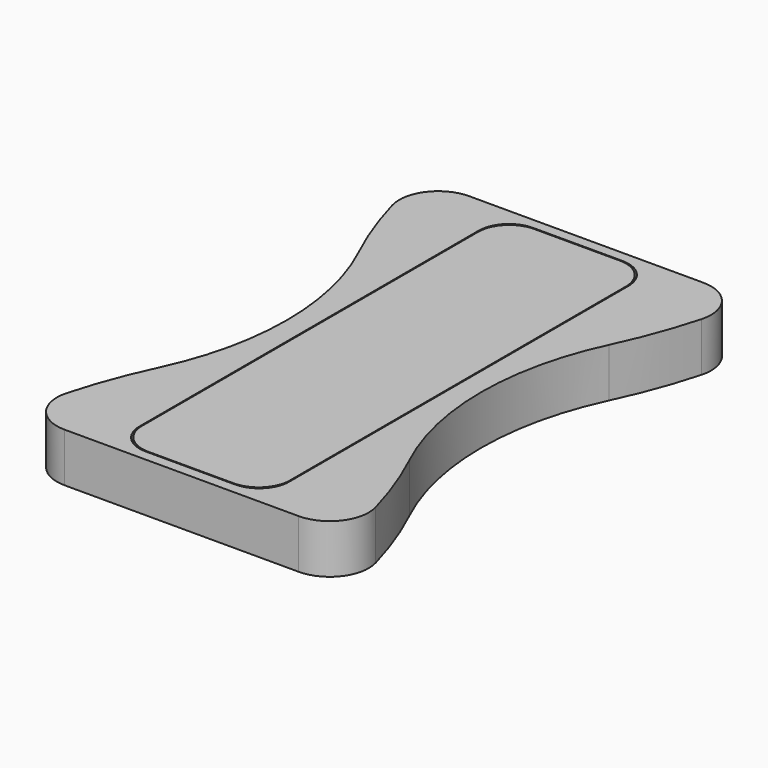
from build123d import *

# Parameters (mm, degrees)
F0_W         = 38
F0_H         = 124
F1_DEPTH     = 6.3
F2_R         = 8
F3_R         = 3
F5_DEPTH     = 6.3
F6_W         = 38.5
F6_H         = 124.5
F7_DEPTH     = 6.15
F8_R         = 7.75
F9_R         = 2.75
F11_DEPTH    = 12.601
F12_T1_DEPTH = 108.1589008266
F13_R        = 10


# Not quite as in the source:
# - a fillet or chamfer that OpenCascade refuses, or shapes differently, is made with other operations: its cross-section is extruded or revolved along the edge and cut away or added


with BuildPart() as f1:
    # F0 (on Top) → F1 (new body)
    with BuildSketch(Plane.XY):
        Rectangle(F0_W, F0_H)
    extrude(amount=F1_DEPTH)

    # F2
    f2_edges = [f1.edges().sort_by_distance(p)[0] for p in [
        (19, 62, 3.15),
        (-19, 62, 3.15),
        (19, -62, 3.15),
        (-19, -62, 3.15),
    ]]
    fillet(f2_edges, radius=F2_R)

    # F3
    f3_edges = [f1.edges().sort_by_distance(p)[0] for p in [
        (0, -62, 0),
        (-16.656854, -59.656854, 0),
        (16.656854, -59.656854, 0),
        (-19, 0, 0),
        (19, 0, 0),
        (-16.656854, 59.656854, 0),
        (16.656854, 59.656854, 0),
        (0, 62, 0),
    ]]
    fillet(f3_edges, radius=F3_R)


with BuildPart() as f5:
    # F4 (on Top) → F5 (new body, symmetric)
    with BuildSketch(Plane.XY):
        with BuildLine():
            Line((19.25, -27.1095328612), (19.25, -62.25))
            Line((19.25, -62.25), (-19.25, -62.25))
            Line((-19.25, -62.25), (-19.25, -27.1095328612))
            ThreePointArc((-19.25, -27.1095328612), (-36.224128699, -42.7724832696), (-42.5, -65))
            Line((-42.5, -65), (42.5, -65))
            ThreePointArc((42.5, -65), (36.224128699, -42.7724832696), (19.25, -27.1095328612))
        make_face()
        with BuildLine():
            ThreePointArc((-42.5, -65), (-36.224128699, -42.7724832696), (-19.25, -27.1095328612))
            Line((-19.25, -27.1095328612), (-19.25, 27.1095328612))
            ThreePointArc((-19.25, 27.1095328612), (-36.224128699, 42.7724832696), (-42.5, 65))
            Line((-42.5, 65), (-42.5, -65))
        make_face()
        with BuildLine():
            Line((19.25, 27.1095328612), (19.25, -27.1095328612))
            ThreePointArc((19.25, -27.1095328612), (36.224128699, -42.7724832696), (42.5, -65))
            Line((42.5, -65), (42.5, 65))
            ThreePointArc((42.5, 65), (36.224128699, 42.7724832696), (19.25, 27.1095328612))
        make_face()
        with BuildLine():
            Line((19.25, 62.25), (19.25, 27.1095328612))
            ThreePointArc((19.25, 27.1095328612), (36.224128699, 42.7724832696), (42.5, 65))
            Line((42.5, 65), (-42.5, 65))
            ThreePointArc((-42.5, 65), (-36.224128699, 42.7724832696), (-19.25, 27.1095328612))
            Line((-19.25, 27.1095328612), (-19.25, 62.25))
            Line((-19.25, 62.25), (19.25, 62.25))
        make_face()
    extrude(amount=F5_DEPTH, both=True)

    # F6 (on face) → F7 (join)
    with BuildSketch(Plane(origin=(0, 0, -6.3), x_dir=(1, 0, 0), z_dir=(0, 0, -1))):
        Rectangle(F6_W, F6_H)
    extrude(amount=-F7_DEPTH)

    # F8
    f8_edges = [f5.edges().sort_by_distance(p)[0] for p in [
        (19.25, -62.25, 3.075),
        (-19.25, -62.25, 3.075),
        (19.25, 62.25, 3.075),
        (-19.25, 62.25, 3.075),
    ]]
    fillet(f8_edges, radius=F8_R)

    # F9
    f9_edges = [f5.edges().sort_by_distance(p)[0] for p in [
        (0, 62.25, -0.15),
        (-16.980078, 59.980078, -0.15),
        (16.980078, 59.980078, -0.15),
        (-19.25, 0, -0.15),
        (19.25, 0, -0.15),
        (-16.980078, -59.980078, -0.15),
        (16.980078, -59.980078, -0.15),
        (0, -62.25, -0.15),
    ]]
    fillet(f9_edges, radius=F9_R)

    # F10 (on face) → F11 (cut, through all)
    with BuildSketch(Plane.XY.offset(6.3)):
        with BuildLine():
            ThreePointArc((-25, 0), (-29.5106391006, 25.6173769149), (-42.5, 48.1534007106))
            Line((-42.5, 48.1534007106), (-42.5, -48.1534007106))
            ThreePointArc((-42.5, -48.1534007106), (-29.5106391006, -25.6173769149), (-25, 0))
        make_face()
        with BuildLine():
            Line((42.5, -48.1534007106), (42.5, 48.1534007106))
            ThreePointArc((42.5, 48.1534007106), (25, 0), (42.5, -48.1534007106))
        make_face()
    extrude(amount=-F11_DEPTH, mode=Mode.SUBTRACT)

    # F12: fillet of radius 125 on 4 edges, made by hand

    # F12_s2 → F12_t1 (cut)
    with BuildSketch(Plane.XY.offset(-54.0794504133)):
        with BuildLine():
            ThreePointArc((32.1962626253, -32.0570303993), (38.4906868537, -48.1711523883), (42.5, -65))
            Line((42.5, -65), (42.5, -48.1534007106))
            ThreePointArc((42.5, -48.1534007106), (36.8333162631, -40.4347630843), (32.1962626253, -32.0570303993))
        make_face()
        with BuildLine():
            ThreePointArc((42.5, 65), (38.4906868537, 48.1711523883), (32.1962626253, 32.0570303993))
            ThreePointArc((32.1962626253, 32.0570303993), (36.8333162631, 40.4347630843), (42.5, 48.1534007106))
            Line((42.5, 48.1534007106), (42.5, 65))
        make_face()
        with BuildLine():
            ThreePointArc((-42.5, -65), (-38.4906868537, -48.1711523883), (-32.1962626253, -32.0570303993))
            ThreePointArc((-32.1962626253, -32.0570303993), (-36.8333162631, -40.4347630843), (-42.5, -48.1534007106))
            Line((-42.5, -48.1534007106), (-42.5, -65))
        make_face()
        with BuildLine():
            ThreePointArc((-32.1962626253, 32.0570303993), (-38.4906868537, 48.1711523883), (-42.5, 65))
            Line((-42.5, 65), (-42.5, 48.1534007106))
            ThreePointArc((-42.5, 48.1534007106), (-36.8333162631, 40.4347630843), (-32.1962626253, 32.0570303993))
        make_face()
    extrude(amount=F12_T1_DEPTH, mode=Mode.SUBTRACT)

    # F13
    f13_edges = [f5.edges().sort_by_distance(p)[0] for p in [
        (-42.5, 65, 0),
        (42.5, 65, 0),
        (-42.5, -65, 0),
        (42.5, -65, 0),
    ]]
    fillet(f13_edges, radius=F13_R)


solid = Compound([f1.part, f5.part])
